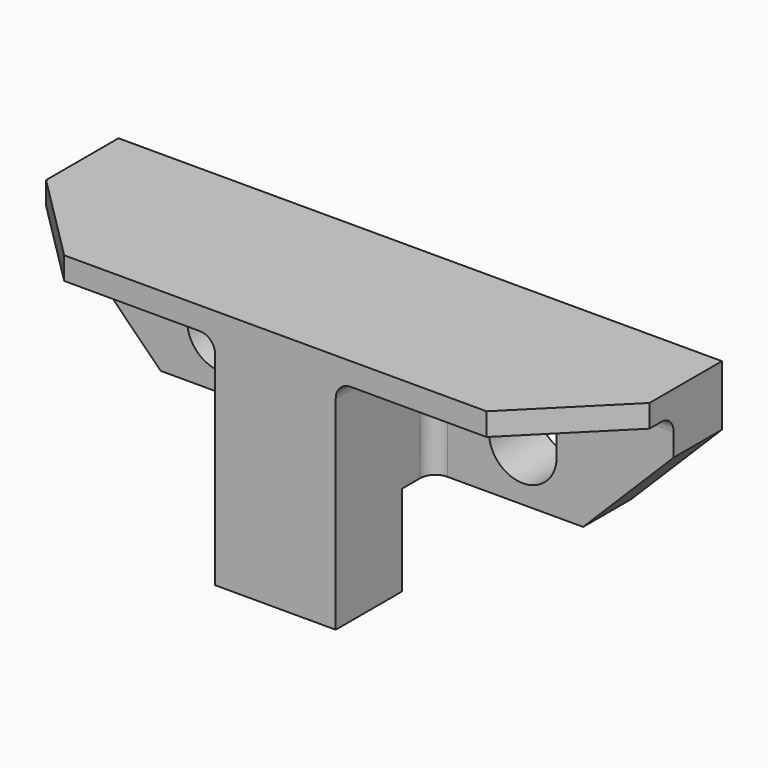
from build123d import *

# Parameters (mm, degrees)
F0_W     = 40
F0_H     = 10
F1_DEPTH = 4
F2_W     = 16
F2_H     = 1.5
F3_DEPTH = 8
F4_W     = 8
F4_H     = 5.5
F5_DEPTH = 6
F6_R     = 1
F7_SIZE  = 6


# Not quite as in the source:
# - a feature names something its author has since deleted; it is built from what else it names


with BuildPart() as f1:
    # F0 (on Front) → F1 (new body)
    with BuildSketch(Plane.XZ):
        Rectangle(F0_W, F0_H)
        with BuildLine():
            Line((-12.25, -1.5), (-12.25, 0.5))
            ThreePointArc((-12.25, 0.5), (-10, 2.75), (-7.75, 0.5))
            Line((-7.75, 0.5), (-7.75, -1.5))
            ThreePointArc((-7.75, -1.5), (-10, -3.75), (-12.25, -1.5))
        make_face(mode=Mode.SUBTRACT)
        with BuildLine():
            ThreePointArc((7.75, 0.5), (10, 2.75), (12.25, 0.5))
            Line((12.25, 0.5), (12.25, -1.5))
            ThreePointArc((12.25, -1.5), (10, -3.75), (7.75, -1.5))
            Line((7.75, -1.5), (7.75, 0.5))
        make_face(mode=Mode.SUBTRACT)
    extrude(amount=F1_DEPTH)

    # F2 (on face) → F3 (join)
    with BuildSketch(Plane.XZ.offset(4)):
        Polygon((4, 5), (-4, 5), (-4, 3.5), (-4, -5), (4, -5), (4, 3.5), align=None)
        with Locations((-12, 4.25)):
            Rectangle(F2_W, F2_H)
        with Locations((12, 4.25)):
            Rectangle(F2_W, F2_H)
    extrude(amount=F3_DEPTH)

    # F4 (on face) → F5 (join)
    with BuildSketch(Plane(origin=(0, 0, -5), x_dir=(1, 0, 0), z_dir=(0, 0, -1))):
        with Locations((0, 9.25)):
            Rectangle(F4_W, F4_H)
    extrude(amount=F5_DEPTH)

    # F6
    f6_edges = [f1.edges().sort_by_distance(p)[0] for p in [
        (4, -4, -0.75),
        (-4, -4, -0.75),
        (-12, -4, 3.5),
        (12, -4, 3.5),
        (4, -8, 3.5),
        (-4, -8, 3.5),
    ]]
    fillet(f6_edges, radius=F6_R)

    # F7
    f7_edges = [f1.edges().sort_by_distance(p)[0] for p in [
        (-20, -12, 4.25),
        (20, -12, 4.25),
        (20, -2, -5),
        (-20, -2, -5),
    ]]
    chamfer(f7_edges, length=F7_SIZE)


solid = f1.part
